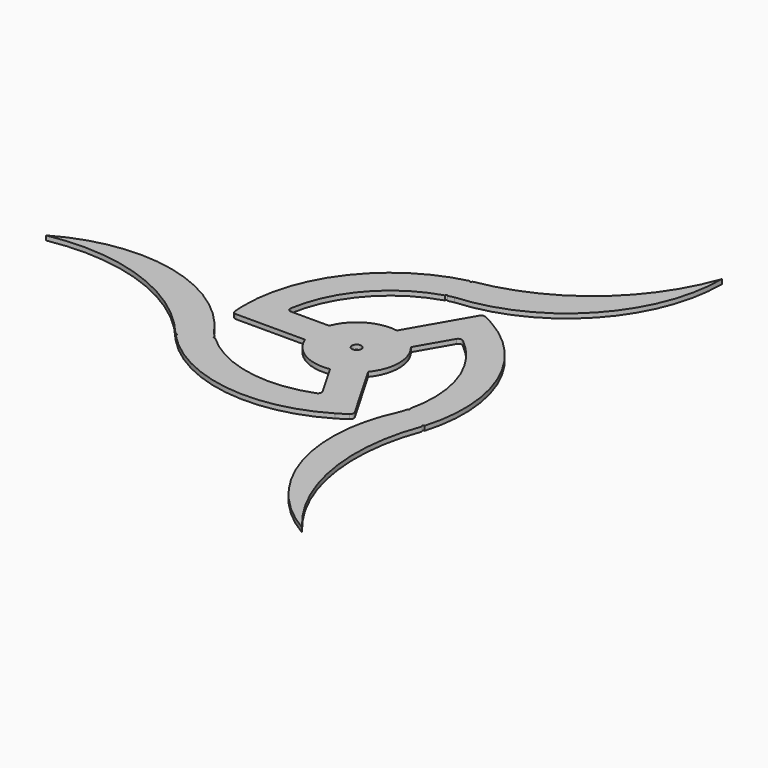
from build123d import *

# Parameters (mm, degrees)
F2_DEPTH        = 1.524
F0_R            = 14.2875
F0_R_2          = 1.5875
F3_COUNT        = 3
F3_ANGLE        = 240
F6_DEPTH        = 240
F6_COPIES_COUNT = 3


# Not quite as in the source:
# - an extrude ends at something that could not be found from the text; its depth is read off the source's solid
# - a pattern or mirror of a feature is missing from the dataset's text; its kind, count and spacing are read off the source's solid
# - a feature names something its author has since deleted; it is built from what else it names


with BuildPart() as f2:
    # F0 (on Top) → F2 (new body)
    with BuildSketch(Plane.XY):
        with BuildLine():
            ThreePointArc((50.8, 90.4875), (31.2220900836, 62.3697318544), (0, 48.26))
            ThreePointArc((0, 48.26), (-27.5567729007, 30.8458733427), (-38.1, 0))
            Line((-38.1, 0), (-27.9404663148, 0.0973411457))
            ThreePointArc((-27.9404663148, 0.0973411457), (-19.5823640029, 24.5502873707), (2.2631606282, 38.3552686068))
            ThreePointArc((2.2631606282, 38.3552686068), (36.7873562722, 54.8729161676), (50.8, 90.4875))
        make_face()
    extrude(amount=F2_DEPTH)


with BuildPart() as f2b:
    # F0 (on Top) → F2, piece 2 (new body)
    with BuildSketch(Plane.XY):
        Circle(F0_R)
        Circle(F0_R_2, mode=Mode.SUBTRACT)
    extrude(amount=F2_DEPTH)


with BuildPart() as f2c:
    # F1 (on face) → F2, piece 3 (new body)
    with BuildSketch(Plane.XY):
        with BuildLine():
            ThreePointArc((-13.3538854365, -5.08), (-14.2875, 0), (-13.3538854365, 5.08))
            Line((-13.3538854365, 5.08), (-26.2094863625, 5.08))
            ThreePointArc((-26.2094863625, 5.08), (-27.1751979909, 5.5251963562), (-27.4638524569, 6.5486597626))
            ThreePointArc((-27.4638524569, 6.5486597626), (-27.8366270568, 3.3329347264), (-27.9404663148, 0.0973411457))
            Line((-27.9404663148, 0.0973411457), (-38.1, 0))
            ThreePointArc((-38.1, 0), (-38.0418102628, -1.963864994), (-37.9049743558, -3.923821038))
            ThreePointArc((-37.9049743558, -3.923821038), (-37.4969244549, -4.7474040533), (-36.6400851229, -5.08))
            Line((-36.6400851229, -5.08), (-13.3538854365, -5.08))
        make_face()
    extrude(amount=F2_DEPTH)


with BuildPart() as f3_1:
    # F3: instance of F2
    add(f2.part.rotate(Axis((0, 0, 0), (0, 0, 1)), 1 * F3_ANGLE / (F3_COUNT - 1)))


with BuildPart() as f3_2:
    # F3: instance of F2
    add(f2.part.rotate(Axis((0, 0, 0), (0, 0, 1)), 2 * F3_ANGLE / (F3_COUNT - 1)))


with BuildPart() as f3_3:
    # F3: instance of F2c
    add(f2c.part.rotate(Axis((0, 0, 0), (0, 0, 1)), 1 * F3_ANGLE / (F3_COUNT - 1)))


with BuildPart() as f3_4:
    # F3: instance of F2c
    add(f2c.part.rotate(Axis((0, 0, 0), (0, 0, 1)), 2 * F3_ANGLE / (F3_COUNT - 1)))


with BuildPart() as f2_1:
    add(f2.part)

    # F4: union F2c, F2b, F3_4, F3_2, F3_3, F3_1
    add(f2c.part)
    add(f2b.part)
    add(f3_4.part)
    add(f3_2.part)
    add(f3_3.part)
    add(f3_1.part)

    # F5 (on face) → F6 (cut, through all)
    with BuildSketch(Plane.XY.offset(1.524)):
        with BuildLine():
            ThreePointArc((0, 48.26), (0.1881613405, 48.2897596913), (0.3762338884, 48.3200754628))
            ThreePointArc((0.3762338884, 48.3200754628), (-0.0732384475, 48.6338945437), (-0.3710948228, 48.1736887464))
            ThreePointArc((-0.3710948228, 48.1736887464), (-0.1856312633, 48.2172048941), (0, 48.26))
        make_face()
        with BuildLine():
            ThreePointArc((-0.3710948228, 48.1736887464), (0.0434388796, 47.8814843943), (0.381, 48.26))
            ThreePointArc((0.381, 48.26), (0.3798066031, 48.2901321135), (0.3762338884, 48.3200754628))
            ThreePointArc((0.3762338884, 48.3200754628), (0.1881613405, 48.2897596913), (0, 48.26))
            ThreePointArc((0, 48.26), (-0.1856312633, 48.2172048941), (-0.3710948228, 48.1736887464))
        make_face()
        with BuildLine():
            ThreePointArc((-0.3651208351, 37.6571250082), (0, 37.7659724968), (0.3661704074, 37.8712351814))
            ThreePointArc((0.3661704074, 37.8712351814), (-0.1070563729, 38.1316225112), (-0.3651208351, 37.6571250082))
        make_face()
    f6 = extrude(amount=-F6_DEPTH, mode=Mode.SUBTRACT)

    # F6_copies: F6 ×3 about axis
    f6_copies_axis = Axis((0, 0, 0), (0, 0, 1))
    for i in range(1, F6_COPIES_COUNT):
        add(f6.rotate(f6_copies_axis, i * 360 / F6_COPIES_COUNT), mode=Mode.SUBTRACT)


solid = f2_1.part
